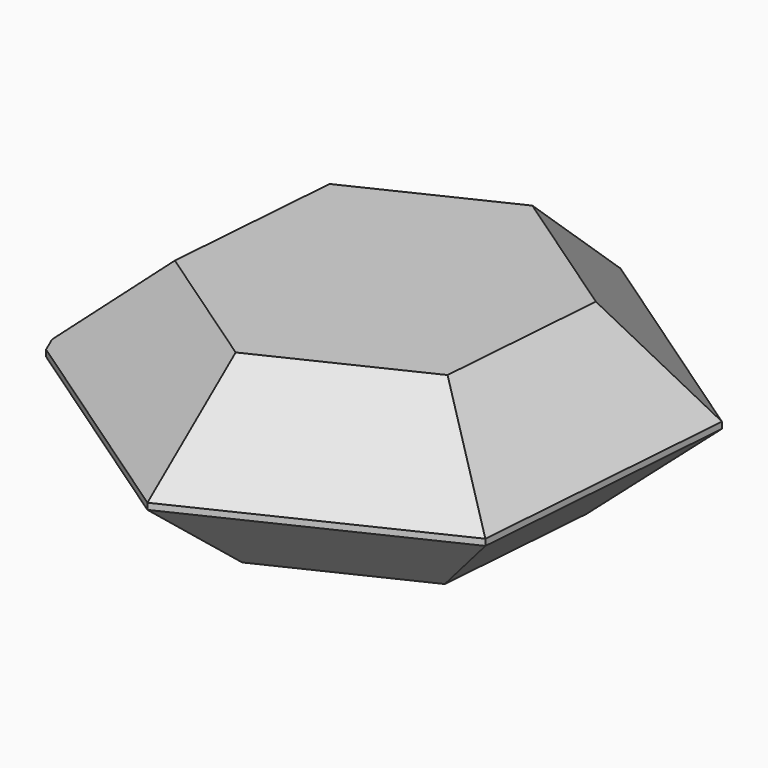
from build123d import *

# Parameters (mm, degrees)
F1_DEPTH     = 10.16
F2_C1_SIZE2  = 10.16
F2_C1_SIZE   = 9.4743532752
F2_C2_SIZE2  = 10.16
F2_C2_SIZE   = 9.4743532752
F2_C3_SIZE2  = 10.16
F2_C3_SIZE   = 9.4743532752
F2_C4_SIZE2  = 9.4743532752
F2_C4_SIZE   = 10.16
F2_C5_SIZE2  = 10.16
F2_C5_SIZE   = 9.4743532752
F2_C6_SIZE2  = 9.4743532752
F2_C6_SIZE   = 10.16
F2_C7_SIZE2  = 10.16
F2_C7_SIZE   = 9.4743532752
F2_C8_SIZE2  = 9.4743532752
F2_C8_SIZE   = 10.16
F2_C9_SIZE2  = 10.16
F2_C9_SIZE   = 9.4743532752
F2_C10_SIZE2 = 9.4743532752
F2_C10_SIZE  = 10.16
F2_C11_SIZE2 = 9.4743532752
F2_C11_SIZE  = 10.16
F2_C12_SIZE2 = 10.16
F2_C12_SIZE  = 9.4743532752


with BuildPart() as f1:
    # F0 (on Top) → F1 (new body, symmetric)
    with BuildSketch(Plane.XY):
        Polygon((-24.2152860866, 16.5479078158), (-26.4385515912, -12.697099003), (-2.2232655046, -29.2450068188), (24.2152860866, -16.5479078158), (26.4385515912, 12.697099003), (2.2232655046, 29.2450068188), align=None)
    extrude(amount=F1_DEPTH, both=True)

    # F2: chamfer of 10.16 x 9.4743532752 on 12 edges, made by hand

    # F2_c1
    f2_c1_edges = [f1.edges().sort_by_distance(p)[0] for p in [
        (-25.3269188389, 1.9254044064, -10.16),
    ]]
    f2_c1_side = f1.faces().sort_by_distance((-25.3269188389, 1.9254044064, -9.9705129345))[0]
    chamfer(f2_c1_edges, length=F2_C1_SIZE, length2=F2_C1_SIZE2, reference=f2_c1_side)

    # F2_c2
    f2_c2_edges = [f1.edges().sort_by_distance(p)[0] for p in [
        (-25.3269188389, 1.9254044064, 10.16),
    ]]
    f2_c2_side = f1.faces().sort_by_distance((-25.3269188389, 1.9254044064, 9.9705129345))[0]
    chamfer(f2_c2_edges, length=F2_C2_SIZE, length2=F2_C2_SIZE2, reference=f2_c2_side)

    # F2_c3
    f2_c3_edges = [f1.edges().sort_by_distance(p)[0] for p in [
        (-5.7082999727, 25.4358771179, -10.16),
    ]]
    f2_c3_side = f1.faces().sort_by_distance((-5.7082999727, 25.4358771179, -9.9705129345))[0]
    chamfer(f2_c3_edges, length=F2_C3_SIZE, length2=F2_C3_SIZE2, reference=f2_c3_side)

    # F2_c4
    f2_c4_edges = [f1.edges().sort_by_distance(p)[0] for p in [
        (-5.7082999727, 25.4358771179, 10.16),
    ]]
    f2_c4_side = f1.faces().sort_by_distance((-5.7082999727, 25.4358771179, 9.9705129345))[0]
    chamfer(f2_c4_edges, length=F2_C4_SIZE, length2=F2_C4_SIZE2, reference=f2_c4_side)

    # F2_c5
    f2_c5_edges = [f1.edges().sort_by_distance(p)[0] for p in [
        (19.1739657652, 17.6614713477, -10.16),
    ]]
    f2_c5_side = f1.faces().sort_by_distance((19.1739657652, 17.6614713477, -9.9705129345))[0]
    chamfer(f2_c5_edges, length=F2_C5_SIZE, length2=F2_C5_SIZE2, reference=f2_c5_side)

    # F2_c6
    f2_c6_edges = [f1.edges().sort_by_distance(p)[0] for p in [
        (18.8471324661, 17.8848181744, 10.16),
    ]]
    f2_c6_side = f1.faces().sort_by_distance((18.8471324661, 17.8848181744, 9.9705129345))[0]
    chamfer(f2_c6_edges, length=F2_C6_SIZE, length2=F2_C6_SIZE2, reference=f2_c6_side)

    # F2_c7
    f2_c7_edges = [f1.edges().sort_by_distance(p)[0] for p in [
        (24.882265738, -7.7744057701, -10.16),
    ]]
    f2_c7_side = f1.faces().sort_by_distance((24.882265738, -7.7744057701, -9.9705129345))[0]
    chamfer(f2_c7_edges, length=F2_C7_SIZE, length2=F2_C7_SIZE2, reference=f2_c7_side)

    # F2_c8
    f2_c8_edges = [f1.edges().sort_by_distance(p)[0] for p in [
        (24.9122731142, -7.3796864169, 10.16),
    ]]
    f2_c8_side = f1.faces().sort_by_distance((24.9122731142, -7.3796864169, 9.9705129345))[0]
    chamfer(f2_c8_edges, length=F2_C8_SIZE, length2=F2_C8_SIZE2, reference=f2_c8_side)

    # F2_c9
    f2_c9_edges = [f1.edges().sort_by_distance(p)[0] for p in [
        (5.7082999727, -25.4358771179, -10.16),
    ]]
    f2_c9_side = f1.faces().sort_by_distance((5.7082999727, -25.4358771179, -9.9705129345))[0]
    chamfer(f2_c9_edges, length=F2_C9_SIZE, length2=F2_C9_SIZE2, reference=f2_c9_side)

    # F2_c10
    f2_c10_edges = [f1.edges().sort_by_distance(p)[0] for p in [
        (6.0651406481, -25.2645045914, 10.16),
    ]]
    f2_c10_side = f1.faces().sort_by_distance((6.0651406481, -25.2645045914, 9.9705129345))[0]
    chamfer(f2_c10_edges, length=F2_C10_SIZE, length2=F2_C10_SIZE2, reference=f2_c10_side)

    # F2_c11
    f2_c11_edges = [f1.edges().sort_by_distance(p)[0] for p in [
        (-14.0040752488, -21.1943997376, 10.16),
    ]]
    f2_c11_side = f1.faces().sort_by_distance((-14.0040752488, -21.1943997376, 9.9705129345))[0]
    chamfer(f2_c11_edges, length=F2_C11_SIZE, length2=F2_C11_SIZE2, reference=f2_c11_side)

    # F2_c12
    f2_c12_edges = [f1.edges().sort_by_distance(p)[0] for p in [
        (-14.3309085479, -20.9710529109, -10.16),
    ]]
    f2_c12_side = f1.faces().sort_by_distance((-14.3309085479, -20.9710529109, -9.9705129345))[0]
    chamfer(f2_c12_edges, length=F2_C12_SIZE, length2=F2_C12_SIZE2, reference=f2_c12_side)


solid = f1.part
